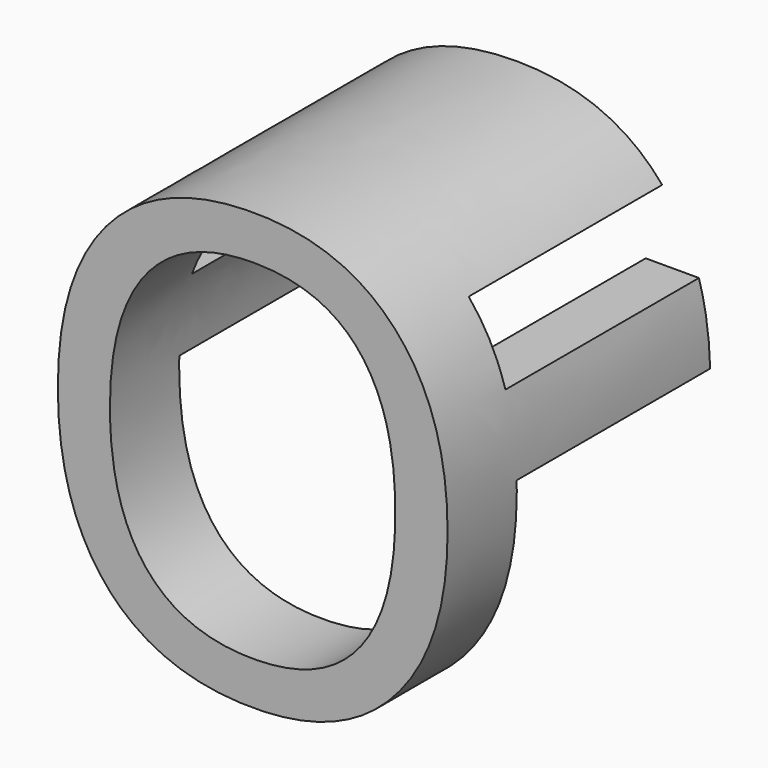
from build123d import *

# Parameters (mm, degrees)
F0_TEXT_SIZE = 68.854747547
F1_DEPTH     = 38.1
F2_W         = 28.0632097274
F2_H         = 8.1204175949
F3_DEPTH     = 50.8
F2_H_2       = 29.6156429686
F4_DEPTH     = 76.2


# Not quite as in the source:
# - Text() gives the source's letters only with a copy of the font that has no kerning and outlines rounded to 1/6400 em; it was checked with that copy


with BuildPart() as f1:
    # F0 (on Front) → F1 (new body)
    with BuildSketch(Plane.XZ):
        with Locations((0.5549453199, -0.7399329916)):
            Text('O', F0_TEXT_SIZE, font='Open Sans', text_align=(TextAlign.LEFT, TextAlign.BOTTOM))
    extrude(amount=F1_DEPTH)

    # F2 (on Right) → F3 (cut)
    with BuildSketch(Plane.YZ):
        with Locations((-14.0316048637, 37.9748977721)):
            Rectangle(F2_W, F2_H)
    extrude(amount=F3_DEPTH, mode=Mode.SUBTRACT)

    # F2 (on Right) → F4 (cut)
    with BuildSketch(Plane.YZ):
        with Locations((-14.0316048637, 10.2699405979)):
            Rectangle(F2_W, F2_H_2)
    extrude(amount=F4_DEPTH, mode=Mode.SUBTRACT)


solid = f1.part
